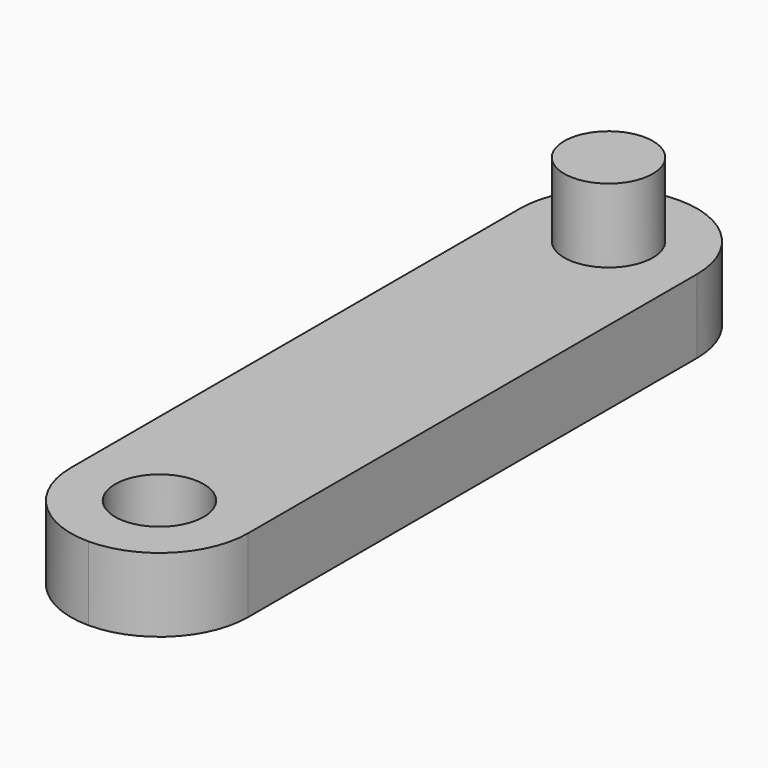
from build123d import *

# Parameters (mm, degrees)
F0_W     = 12
F0_H     = 50
F0_R     = 3
F1_DEPTH = 5
F2_R     = 5.99999
F3_DEPTH = 10


# Not quite as in the source:
# - a fillet or chamfer is up to 0.001 mm smaller than in the source, because OpenCascade refuses the exact size


with BuildPart() as f1:
    # F0 (on Top) → F1 (new body)
    with BuildSketch(Plane.XY):
        with Locations((-0.8723753854, -8.5783358663)):
            Rectangle(F0_W, F0_H)
        with Locations((-0.8723753854, -27.5783358663)):
            Circle(F0_R, mode=Mode.SUBTRACT)
        with Locations((-0.8723753854, 10.4216641337)):
            Circle(F0_R, mode=Mode.SUBTRACT)
    extrude(amount=F1_DEPTH)

    # F2 (radius 6 in the source; OpenCascade refuses exactly that, so slightly less here)
    f2_edges = [f1.edges().sort_by_distance(p)[0] for p in [
        (-6.872375, 16.421664, 2.5),
        (5.127625, 16.421664, 2.5),
        (5.127625, -33.578336, 2.5),
        (-6.872375, -33.578336, 2.5),
    ]]
    fillet(f2_edges, radius=F2_R)

    # F0 (on Top) → F3 (join)
    with BuildSketch(Plane.XY):
        with Locations((-0.8723753854, 10.4216641337)):
            Circle(F0_R)
    extrude(amount=F3_DEPTH)


solid = f1.part
